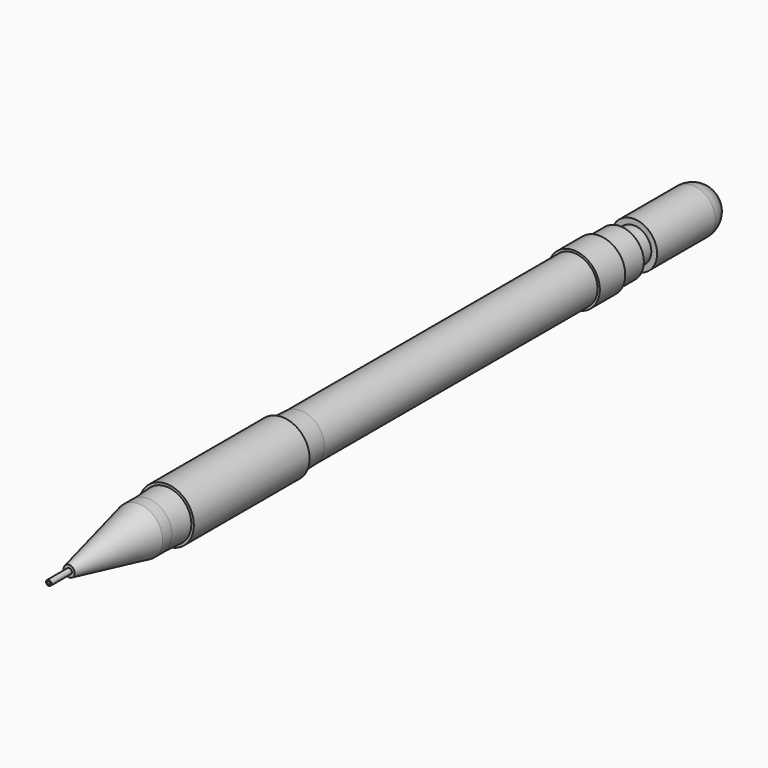
from build123d import *

# Parameters (mm, degrees)
F0_R      = 4.11
F1_DEPTH  = 69
F2_R      = 3
F3_DEPTH  = 3
F4_R      = 4
F5_DEPTH  = 16.6
F6_R      = 4
F7_R      = 4.11
F8_DEPTH  = 4
F8_TAPER  = -3
F9_R      = 4.75
F10_DEPTH = 25
F11_R     = 4.3195
F12_DEPTH = 4
F12_TAPER = 3
F15_R     = 4.15
F16_DEPTH = 2
F17_R     = 4.15
F18_DEPTH = 15
F18_TAPER = 12
F19_R     = 0.47
F20_DEPTH = 4.4
F21_R     = 0.25
F22_DEPTH = 25
F25_R     = 4.5
F25_R_2   = 4.11
F26_DEPTH = 5.5


# Not quite as in the source:
# - a feature of the source that left no trace in its solid (it failed there, or was rolled back) is left out


with BuildPart() as f1:
    # F0 (on Front) → F1 (new body)
    with BuildSketch(Plane.XZ):
        Circle(F0_R)
    extrude(amount=F1_DEPTH)


with BuildPart() as f3:
    # F2 (on face) → F3 (new body)
    with BuildSketch(Plane(origin=(0, 0, 0), x_dir=(-1, 0, 0), z_dir=(0, 1, 0))):
        Circle(F2_R)
    extrude(amount=F3_DEPTH)


with BuildPart() as f5:
    # F4 (on face) → F5 (new body)
    with BuildSketch(Plane(origin=(0, 3, 0), x_dir=(-1, 0, 0), z_dir=(0, 1, 0))):
        Circle(F4_R)
    extrude(amount=F5_DEPTH)

    # F6
    f6_edges = [f5.edges().sort_by_distance(p)[0] for p in [
        (4, 19.6, 0),
    ]]
    fillet(f6_edges, radius=F6_R)


with BuildPart() as f8:
    # F7 (on face) → F8 (new body)
    with BuildSketch(Plane.XZ.offset(69)):
        Circle(F7_R)
    extrude(amount=F8_DEPTH, taper=F8_TAPER)

    # F9 (on face) → F10 (join)
    with BuildSketch(Plane.XZ.offset(73)):
        Circle(F9_R)
    extrude(amount=F10_DEPTH)

    # F11 (on face) → F12 (join)
    with BuildSketch(Plane.XZ.offset(98)):
        Circle(F11_R)
    extrude(amount=F12_DEPTH, taper=F12_TAPER)


with BuildPart() as f16:
    # F15 (on face) → F16 (new body)
    with BuildSketch(Plane.XZ.offset(102)):
        Circle(F15_R)
    extrude(amount=F16_DEPTH)

    # F17 (on face) → F18 (join)
    with BuildSketch(Plane.XZ.offset(104)):
        Circle(F17_R)
    extrude(amount=F18_DEPTH, taper=F18_TAPER)

    # F19 (on face) → F20 (join)
    with BuildSketch(Plane.XZ.offset(119)):
        Circle(F19_R)
    extrude(amount=F20_DEPTH)

    # F21 (on face) → F22 (cut)
    with BuildSketch(Plane.XZ.offset(123.4)):
        Circle(F21_R)
    extrude(amount=-F22_DEPTH, mode=Mode.SUBTRACT)


with BuildPart() as f26:
    # F25 (on offset) → F26 (new body)
    with BuildSketch(Plane(origin=(0, -4.5, 0), x_dir=(-1, 0, 0), z_dir=(0, 1, 0))):
        Circle(F25_R)
        Circle(F25_R_2, mode=Mode.SUBTRACT)
    extrude(amount=-F26_DEPTH)


solid = Compound([f1.part, f3.part, f5.part, f8.part, f16.part, f26.part])
